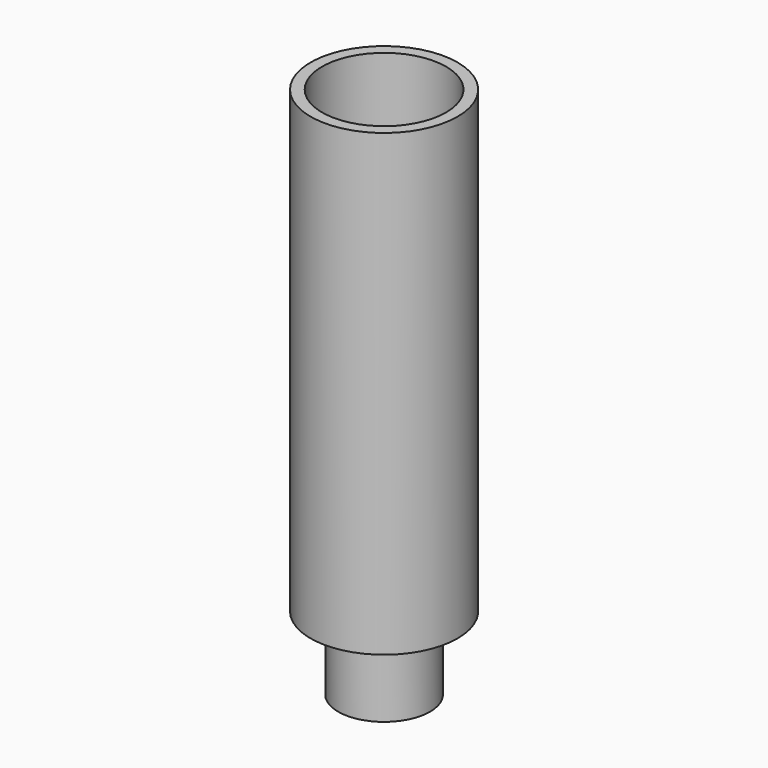
from build123d import *

# Parameters (mm, degrees)
F0_R        = 5
F0_R_2      = 3.5
F1_DEPTH    = 8
F2_R        = 8
F2_R_2      = 6.75
F2_R_3      = 5
F2_R_4      = 3.5
F2_R_5      = 2
F2_R_6      = 1.5
F3_DEPTH    = 1
F4_DEPTH    = 50
F5_DEPTH    = 25
F6_S5_R     = 1.5
F6_T6_DEPTH = 8
F7_R        = 2
F9_R        = 2


# Not quite as in the source:
# - a fillet or chamfer that OpenCascade refuses, or shapes differently, is made with other operations: its cross-section is extruded or revolved along the edge and cut away or added


with BuildPart() as f1:
    # F0 (on Top) → F1 (new body)
    with BuildSketch(Plane.XY):
        Circle(F0_R)
        Circle(F0_R_2, mode=Mode.SUBTRACT)
    extrude(amount=F1_DEPTH)

    # F2 (on face) → F3 (join)
    with BuildSketch(Plane.XY.offset(8)):
        Circle(F2_R)
        Circle(F2_R_2, mode=Mode.SUBTRACT)
        Circle(F2_R_2)
        Circle(F2_R_3, mode=Mode.SUBTRACT)
        Circle(F2_R_3)
        Circle(F2_R_4, mode=Mode.SUBTRACT)
        Circle(F2_R_4)
        Circle(F2_R_5, mode=Mode.SUBTRACT)
        Circle(F2_R_5)
        Circle(F2_R_6, mode=Mode.SUBTRACT)
    extrude(amount=F3_DEPTH)

    # F2 (on face) → F4 (join)
    with BuildSketch(Plane.XY.offset(8)):
        Circle(F2_R)
        Circle(F2_R_2, mode=Mode.SUBTRACT)
    extrude(amount=F4_DEPTH)

    # F2 (on face) → F5 (join)
    with BuildSketch(Plane.XY.offset(8)):
        Circle(F2_R_5)
        Circle(F2_R_6, mode=Mode.SUBTRACT)
    extrude(amount=F5_DEPTH)

    # F6: chamfer of 8 x 3 on 1 edges, made by hand


with BuildPart() as f6_tool2:
    # F6_s3 → F6_t4 (revolve)
    with BuildSketch(Plane.XZ):
        Polygon((0.5, 8), (3.5, 0), (3.5, 8), align=None)
    revolve(axis=Axis((0, 0, 8), (0, 0, 1)))

    # F6_s5 → F6_t6 (cut, symmetric)
    with BuildSketch(Plane.XY.offset(4)):
        Circle(F6_S5_R)
    extrude(amount=F6_T6_DEPTH, both=True, mode=Mode.SUBTRACT)

    split(bisect_by=Plane.XY, keep=Keep.TOP)


with BuildPart() as f1_1:
    add(f1.part)

    # F6_t1: union F6_tool2
    add(f6_tool2.part)

    # F7
    f7_edges = [f1_1.edges().sort_by_distance(p)[0] for p in [
        (-2, 0, 9),
    ]]
    fillet(f7_edges, radius=F7_R)

    # F8: chamfer of 1 x 10 on 1 edges, made by hand

    # F8_s1 → F8_t2 (revolve, cut)
    with BuildSketch(Plane.XZ):
        Polygon((2, 23), (1, 33), (2, 33), align=None)
    revolve(axis=Axis((0, 0, 33), (0, 0, 1)), mode=Mode.SUBTRACT)

    # F9
    f9_edges = [f1_1.edges().sort_by_distance(p)[0] for p in [
        (-6.75, 0, 9),
    ]]
    fillet(f9_edges, radius=F9_R)


solid = f1_1.part
